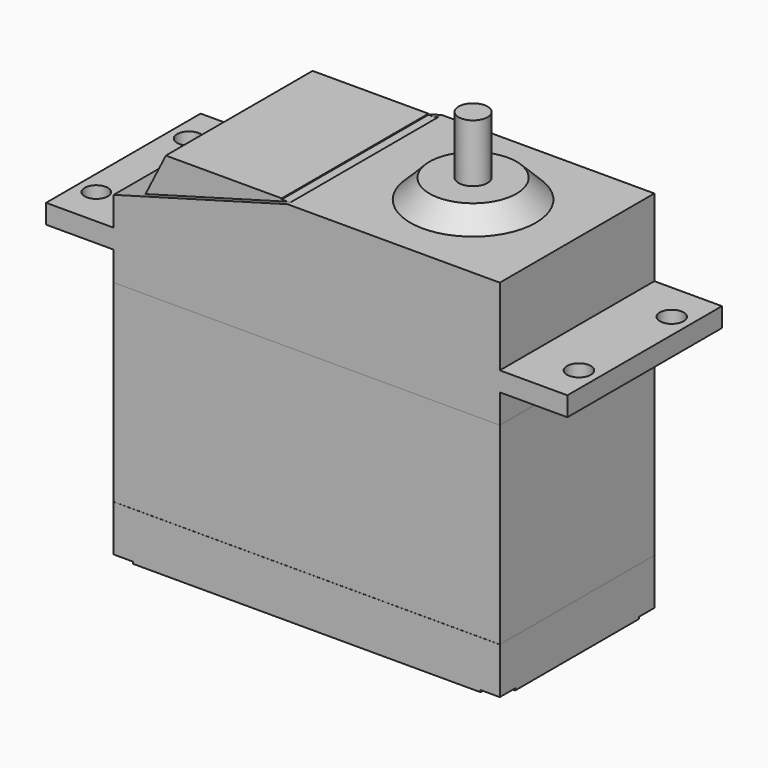
from build123d import *

# Parameters (mm, degrees)
F0_W      = 7
F0_H      = 2
F1_DEPTH  = 20.01
F0_W_2    = 40
F0_H_2    = 5
F0_H_3    = 20
F2_DEPTH  = 20
F3_R      = 1.2382162301
F3_R_2    = 1.2382178276
F3_R_3    = 1.2002117001
F3_R_4    = 1.2382157204
F4_DEPTH  = 5
F5_DEPTH  = 19.5
F6_DEPTH  = 0.5
F7_W      = 1
F7_H      = 19
F8_DEPTH  = 0.1
F7_R      = 1.5
F9_DEPTH  = 8
F7_R_2    = 6.5
F10_DEPTH = 2
F11_SIZE  = 1.99999
F13_DEPTH = 0.2


# Not quite as in the source:
# - a fillet or chamfer is up to 0.001 mm smaller than in the source, because OpenCascade refuses the exact size


with BuildPart() as f1:
    # F0 (on Front) → F1 (new body)
    with BuildSketch(Plane.XZ):
        Polygon((-99.4207011163, 11.8651846424), (-99.4207011163, 8.8651846424), (-59.4207011163, 8.8651846424), (-59.4207011163, 11.8651846424), (-59.4207011163, 13.8651846424), (-59.4207011163, 21.8651846424), (-81.4207011163, 21.8651846424), (-96.5301473874, 17.6681162337), (-99.4207011163, 16.8651846424), (-99.4207011163, 13.8651846424), align=None)
        with Locations((-102.9207011163, 12.8651846424)):
            Rectangle(F0_W, F0_H)
        with Locations((-55.9207011163, 12.8651846424)):
            Rectangle(F0_W, F0_H)
    extrude(amount=F1_DEPTH)

    # F3 (on face) → F4 (cut)
    with BuildSketch(Plane.XY.offset(13.8651846424)):
        with Locations((-54.4207011163, -4)):
            Circle(F3_R)
        with Locations((-54.4207011163, -16.01)):
            Circle(F3_R_2)
        with Locations((-104.4207011163, -16.01)):
            Circle(F3_R_3)
        with Locations((-104.4207011163, -4)):
            Circle(F3_R_4)
    extrude(amount=-F4_DEPTH, mode=Mode.SUBTRACT)

    # F0 (on Front) → F5 (join)
    with BuildSketch(Plane.XZ):
        Polygon((-94.4207011163, 21.8651846424), (-96.5301473874, 17.6681162337), (-81.4207011163, 21.8651846424), align=None)
    extrude(amount=F5_DEPTH)

    # F0 (on Front) → F6 (cut)
    with BuildSketch(Plane.XZ):
        Polygon((-94.4207011163, 21.8651846424), (-96.5301473874, 17.6681162337), (-81.4207011163, 21.8651846424), align=None)
    extrude(amount=F6_DEPTH, mode=Mode.SUBTRACT)

    # F7 (on face) → F8 (cut)
    with BuildSketch(Plane.XY.offset(21.8651846424)):
        with Locations((-81.9207011163, -10)):
            Rectangle(F7_W, F7_H)
    extrude(amount=-F8_DEPTH, mode=Mode.SUBTRACT)

    # F7 (on face) → F9 (join)
    with BuildSketch(Plane.XY.offset(21.8651846424)):
        with Locations((-70.1991021633, -10)):
            Circle(F7_R)
    extrude(amount=F9_DEPTH)

    # F7 (on face) → F10 (join)
    with BuildSketch(Plane.XY.offset(21.8651846424)):
        with Locations((-70.1991021633, -10)):
            Circle(F7_R_2)
        with Locations((-70.1991021633, -10)):
            Circle(F7_R, mode=Mode.SUBTRACT)
    extrude(amount=F10_DEPTH)

    # F11 (size 2 in the source; OpenCascade refuses exactly that, so slightly less here)
    f11_edges = [f1.edges().sort_by_distance(p)[0] for p in [
        (-76.699102, -10, 23.865185),
    ]]
    chamfer(f11_edges, length=F11_SIZE)


with BuildPart() as f1b:
    # F0 (on Front) → F1, piece 2 (new body)
    with BuildSketch(Plane.XZ):
        with Locations((-79.4207011163, -13.6348153576)):
            Rectangle(F0_W_2, F0_H_2)
    extrude(amount=F1_DEPTH)

    # F12 (on face) → F13 (cut)
    with BuildSketch(Plane(origin=(0, 0, -16.1348153576), x_dir=(1, 0, 0), z_dir=(0, 0, -1))):
        with BuildLine():
            Line((-59.4207011163, 0), (-59.4207011163, 2))
            ThreePointArc((-59.4207011163, 2), (-60.8349146787, 1.4142135624), (-61.4207011163, 0))
            Line((-61.4207011163, 0), (-59.4207011163, 0))
        make_face()
        with BuildLine():
            ThreePointArc((-61.4207011163, 20.01), (-60.8349146787, 18.5957864376), (-59.4207011163, 18.01))
            Line((-59.4207011163, 18.01), (-59.4207011163, 20.01))
            Line((-59.4207011163, 20.01), (-61.4207011163, 20.01))
        make_face()
        with BuildLine():
            ThreePointArc((-99.4207011163, 18.01), (-98.006487554, 18.5957864376), (-97.4207011163, 20.01))
            Line((-97.4207011163, 20.01), (-99.4207011163, 20.01))
            Line((-99.4207011163, 20.01), (-99.4207011163, 18.01))
        make_face()
        with BuildLine():
            Line((-99.4207011163, 0), (-97.4207011163, 0))
            ThreePointArc((-97.4207011163, 0), (-98.006487554, 1.4142135624), (-99.4207011163, 2))
            Line((-99.4207011163, 2), (-99.4207011163, 0))
        make_face()
    extrude(amount=-F13_DEPTH, mode=Mode.SUBTRACT)


with BuildPart() as f2:
    # F0 (on Front) → F2 (new body)
    with BuildSketch(Plane.XZ):
        with Locations((-79.4207011163, -1.1348153576)):
            Rectangle(F0_W_2, F0_H_3)
    extrude(amount=F2_DEPTH)


solid = Compound([f1.part, f1b.part, f2.part])
